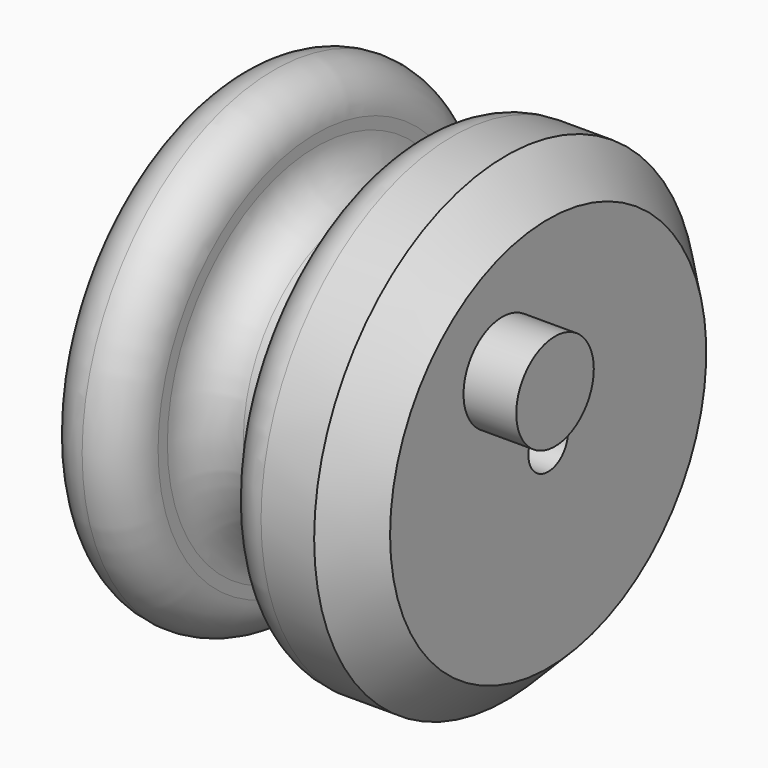
from build123d import *

# Parameters (mm, degrees)
F2_R     = 10.16
F3_R     = 10.15999
F4_SIZE  = 10.16
F5_R     = 11.6722711508
F6_DEPTH = 12.7


# Not quite as in the source:
# - a fillet or chamfer is up to 0.001 mm smaller than in the source, because OpenCascade refuses the exact size


with BuildPart() as f1:
    # F0 (on Top) → F1 (revolve)
    with BuildSketch(Plane.XY):
        Polygon((13.2833082484, -5.9688821161), (-62.9155904868, -5.5592096381), (-62.9155904868, -57.7605935774), (-42.5955904868, -57.7605935774), (-42.5955904868, -34.6378330882), (-19.8231756745, -34.6378330882), (-19.8231756745, -57.7605935774), (13.2833082484, -57.7605935774), align=None)
    revolve(axis=Axis((2.649359405, 0, 0), (1, 0, 0)))

    # F2
    f2_edges = [f1.edges().sort_by_distance(p)[0] for p in [
        (-62.91559, 57.760594, 0),
    ]]
    fillet(f2_edges, radius=F2_R)

    # F3 (radius 10.16 in the source; OpenCascade refuses exactly that, so slightly less here)
    f3_edges = [f1.edges().sort_by_distance(p)[0] for p in [
        (-19.823176, 57.760594, 0),
        (-19.823176, 34.637833, 0),
        (-42.59559, 57.760594, 0),
        (-52.75559, 57.760594, 0),
        (-42.59559, 34.637833, 0),
    ]]
    fillet(f3_edges, radius=F3_R)

    # F4
    f4_edges = [f1.edges().sort_by_distance(p)[0] for p in [
        (13.283308, 57.760594, 0),
    ]]
    chamfer(f4_edges, length=F4_SIZE)

    # F5 (on face) → F6 (join)
    with BuildSketch(Plane.YZ.offset(13.2833082484)):
        with Locations((-13.8126136735, 20.8303108811)):
            Circle(F5_R)
    extrude(amount=F6_DEPTH)


solid = f1.part
